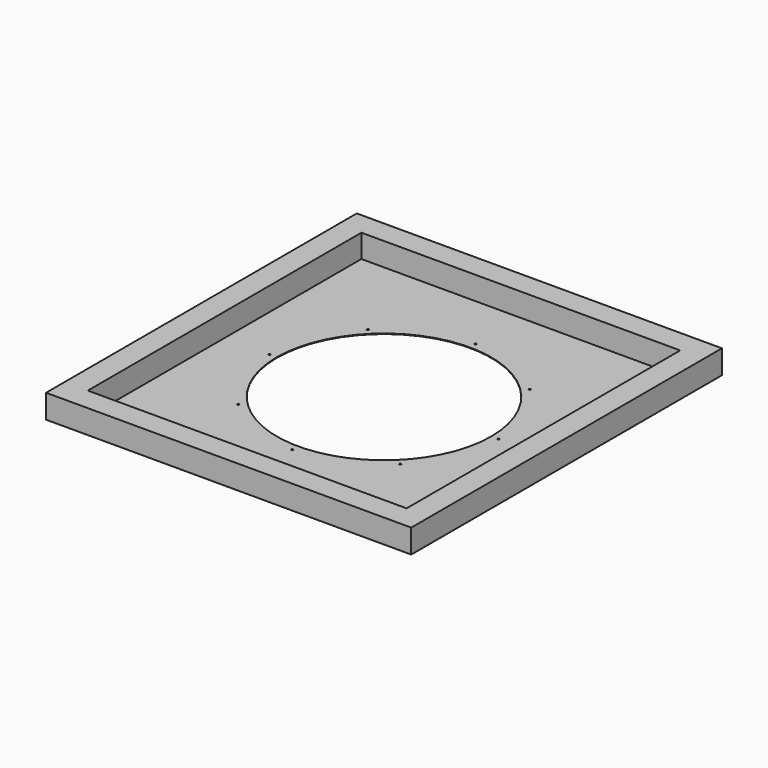
from build123d import *

# Parameters (mm, degrees)
F1_DEPTH = 40
F0_R     = 185
F2_DEPTH = 1
F3_D     = 3.3
F3_DEPTH = 50
F3_TIP   = 0.9914200214
F4_D     = 5.5


# Not quite as in the source:
# - a feature names something its author has since deleted; it is built from what else it names


with BuildPart() as f1:
    # F0 (on Top) → F1 (new body)
    with BuildSketch(Plane.XY):
        Polygon((-275, -295), (-275, 295), (-275, 335), (-315, 335), (-315, -335), (-275, -335), align=None)
        Polygon((-275, 295), (-24.79, 295), (275, 295), (275, 335), (-275, 335), align=None)
        Polygon((275, 335), (275, 295), (275, -295), (275, -325), (275, -335), (315, -335), (315, 335), align=None)
        Polygon((275, -325), (275, -295), (-275, -295), (-275, -335), (0, -335), (275, -335), align=None)
    extrude(amount=F1_DEPTH)


with BuildPart() as f2:
    # F0 (on Top) → F2 (new body)
    with BuildSketch(Plane.XY):
        Polygon((275, 295), (-24.79, 295), (-275, 295), (-275, -295), (275, -295), align=None)
        Circle(F0_R, mode=Mode.SUBTRACT)
        Polygon((-275, 295), (-24.79, 295), (275, 295), (275, 335), (-275, 335), align=None)
        Polygon((275, 335), (275, 295), (275, -295), (275, -325), (275, -335), (315, -335), (315, 335), align=None)
        Polygon((-275, -295), (-275, 295), (-275, 335), (-315, 335), (-315, -335), (-275, -335), align=None)
        Polygon((275, -325), (275, -295), (-275, -295), (-275, -335), (0, -335), (275, -335), align=None)
    extrude(amount=-F2_DEPTH)

    # F3
    with Locations(Plane.XY):
        with Locations((0, 197.5), (139.6535892843, 139.6535892843), (197.5, 0), (139.6535892843, -139.6535892843), (0, -197.5), (-139.6535892843, -139.6535892843), (-139.6535892843, 139.6535892843), (-197.5, 0)):
            Hole(F3_D / 2, depth=F3_DEPTH)
            with Locations((0, 0, -(F3_DEPTH + F3_TIP / 2))):  # 118° drill point
                Cone(0, F3_D / 2, F3_TIP, mode=Mode.SUBTRACT)

    # F4 (through all)
    with Locations(Plane.XY):
        with Locations((295.01, -315), (295.01, -105), (295.01, 105), (295.01, 315), (98.34, 315), (-98.33, 315), (-295, 315), (-295, 105), (-295, -105), (-295, -315), (-98.33, -315), (98.34, -315)):
            Hole(F4_D / 2)


solid = Compound([f1.part, f2.part])
